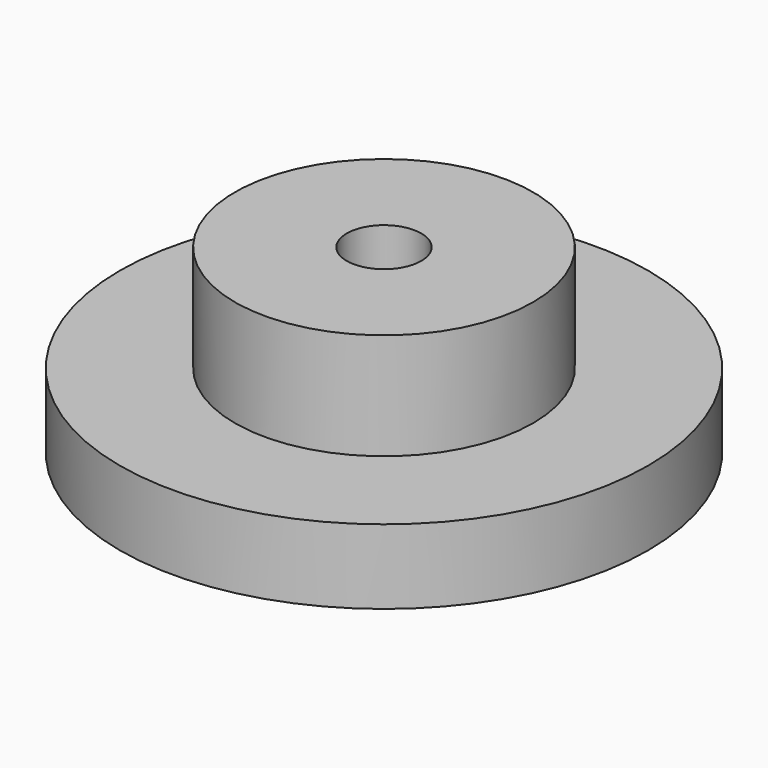
from build123d import *

# Parameters (mm, degrees)
F0_R     = 9
F1_DEPTH = 2.54
F2_R     = 5.08
F3_DEPTH = 3.6285714286
F4_R     = 1.27
F5_DEPTH = 3.6285714286


# Not quite as in the source:
# - a length typed as a fraction of an inch, garbled in the dataset ("3 / 203.2 mm" for 3/8 in), is restored


with BuildPart() as f1:
    # F0 (on Top) → F1 (new body)
    with BuildSketch(Plane.XY):
        Circle(F0_R)
    extrude(amount=F1_DEPTH)

    # F2 (on face) → F3 (join)
    with BuildSketch(Plane.XY.offset(2.54)):
        Circle(F2_R)
    extrude(amount=F3_DEPTH)

    # F4 (on face) → F5 (cut)
    with BuildSketch(Plane.XY.offset(6.1685714286)):
        Circle(F4_R)
    extrude(amount=-F5_DEPTH, mode=Mode.SUBTRACT)


solid = f1.part
